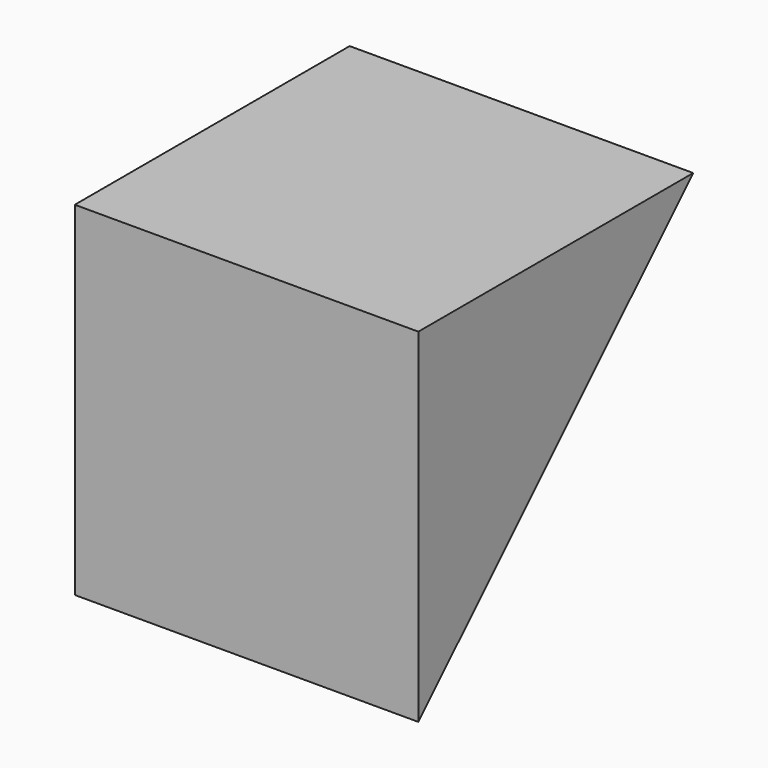
from build123d import *

# Parameters (mm, degrees)
F0_W     = 10
F0_H     = 10
F1_DEPTH = 10
F2_SIZE  = 9.99999


# Not quite as in the source:
# - a fillet or chamfer is up to 0.001 mm smaller than in the source, because OpenCascade refuses the exact size


with BuildPart() as f1:
    # F0 (on Top) → F1 (new body)
    with BuildSketch(Plane.XY):
        Rectangle(F0_W, F0_H)
    extrude(amount=F1_DEPTH)

    # F2 (size 10 in the source; OpenCascade refuses exactly that, so slightly less here)
    f2_edges = [f1.edges().sort_by_distance(p)[0] for p in [
        (0, 5, 0),
    ]]
    chamfer(f2_edges, length=F2_SIZE)


solid = f1.part
